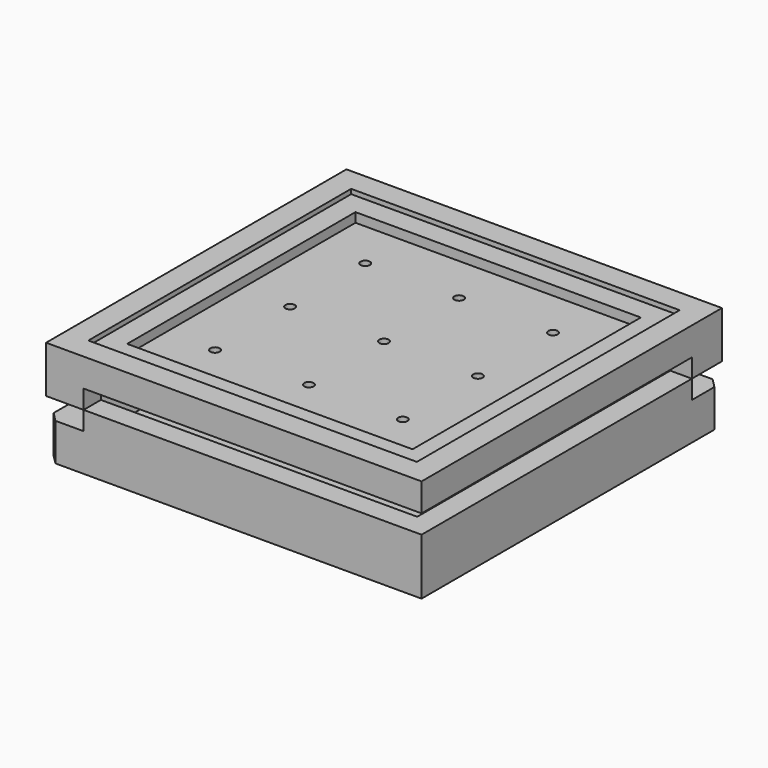
from build123d import *

# Parameters (mm, degrees)
F0_W      = 40
F0_H      = 40
F1_DEPTH  = 6
F4_W      = 40
F4_H      = 40
F5_DEPTH  = 3
F2_W      = 35.4
F2_H      = 35.4
F6_DEPTH  = 1
F6_FACE_W = 35.4
F6_FACE_H = 35.4
F7_DEPTH  = 3
F7_TAPER  = 10
F9_W      = 35.4
F9_H      = 35.4
F10_DEPTH = 1
F11_T     = -2.5
F12_R     = 0.5
F13_DEPTH = 2.5
F13_TAPER = -5
F14_SIZE  = 1
F17_W     = 4
F17_H     = 4
F18_DEPTH = 2
F19_W     = 35.4
F19_H     = 35.4
F20_DEPTH = 25
F15_W     = 4
F15_H     = 4
F21_DEPTH = 2


with BuildPart() as f1:
    # F0 (on Top) → F1 (new body)
    with BuildSketch(Plane.XY):
        with Locations((20, 20)):
            Rectangle(F0_W, F0_H)
    extrude(amount=F1_DEPTH)

    # F2 (on face) → F6 (cut)
    with BuildSketch(Plane.XY.offset(6)):
        with Locations((20, 20)):
            Rectangle(F2_W, F2_H)
    extrude(amount=-F6_DEPTH, mode=Mode.SUBTRACT)

    # F6_face (on face) → F7 (cut)
    with BuildSketch(Plane(origin=(20, 20, 5), x_dir=(1, 0, 0), z_dir=(0, 0, 1))):
        Rectangle(F6_FACE_W, F6_FACE_H)
    extrude(amount=-F7_DEPTH, taper=F7_TAPER, mode=Mode.SUBTRACT)

    # F14
    f14_edges = [f1.edges().sort_by_distance(p)[0] for p in [
        (0, 0, 3),
        (40, 40, 3),
    ]]
    chamfer(f14_edges, length=F14_SIZE)

    # F15 (on face) → F21 (cut)
    with BuildSketch(Plane.XY.offset(6)):
        with Locations((2, 2)):
            Rectangle(F15_W, F15_H)
        with Locations((38, 38)):
            Rectangle(F15_W, F15_H)
    extrude(amount=-F21_DEPTH, mode=Mode.SUBTRACT)


with BuildPart() as f5:
    # F4 (on offset) → F5 (new body)
    with BuildSketch(Plane.XY.offset(11)):
        with Locations((20, 20)):
            Rectangle(F4_W, F4_H)
    extrude(amount=-F5_DEPTH)

    # F9 (on face) → F10 (join)
    with BuildSketch(Plane(origin=(0, 0, 8), x_dir=(1, 0, 0), z_dir=(0, 0, -1))):
        with Locations((20, -20)):
            Rectangle(F9_W, F9_H)
    extrude(amount=F10_DEPTH)

    # F11
    f11_openings = [f5.faces().sort_by_distance(p)[0] for p in [
        (20, 20, 11),
    ]]
    offset(amount=F11_T, openings=f11_openings, kind=Kind.INTERSECTION)

    # F12 (on face) → F13 (cut, through all)
    with BuildSketch(Plane.XY.offset(9.5)):
        with Locations((10, 30)):
            Circle(F12_R)
        with Locations((20, 30)):
            Circle(F12_R)
        with Locations((30, 30)):
            Circle(F12_R)
        with Locations((10, 20)):
            Circle(F12_R)
        with Locations((10, 10)):
            Circle(F12_R)
        with Locations((20, 20)):
            Circle(F12_R)
        with Locations((20, 10)):
            Circle(F12_R)
        with Locations((30, 20)):
            Circle(F12_R)
        with Locations((30, 10)):
            Circle(F12_R)
    extrude(amount=-F13_DEPTH, taper=F13_TAPER, mode=Mode.SUBTRACT)

    # F17 (on face) → F18 (join)
    with BuildSketch(Plane(origin=(0, 0, 8), x_dir=(1, 0, 0), z_dir=(0, 0, -1))):
        with Locations((2, -2)):
            Rectangle(F17_W, F17_H)
        with Locations((38, -38)):
            Rectangle(F17_W, F17_H)
    extrude(amount=F18_DEPTH)

    # F19 (on face) → F20 (cut)
    with BuildSketch(Plane(origin=(0, 0, 7), x_dir=(1, 0, 0), z_dir=(0, 0, -1))):
        with Locations((20, -20)):
            Rectangle(F19_W, F19_H)
    extrude(amount=F20_DEPTH, mode=Mode.SUBTRACT)


solid = Compound([f1.part, f5.part])
